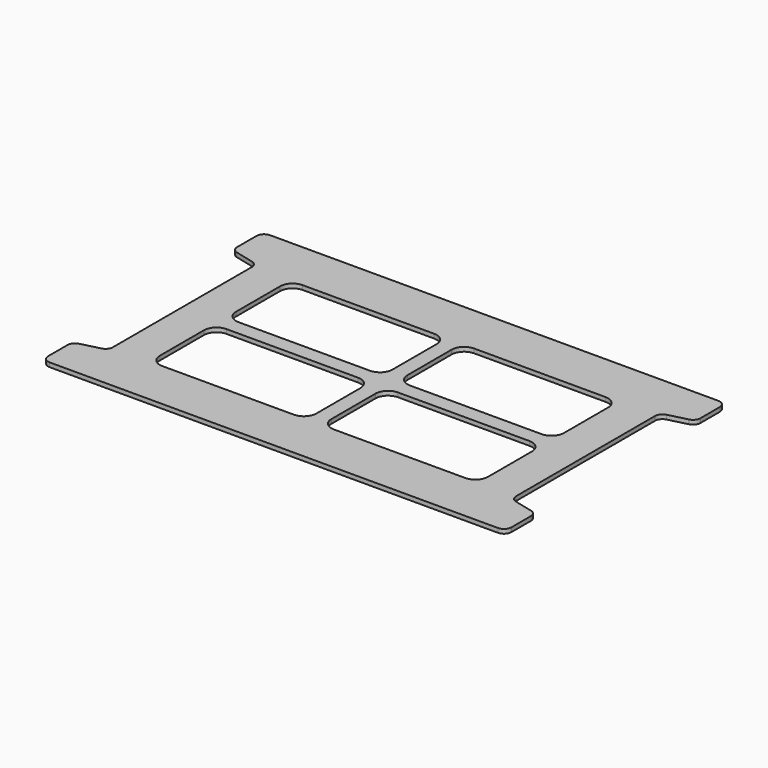
from build123d import *

# Parameters (mm, degrees)
F1_DEPTH = 1.7
F2_R     = 3
F3_W     = 62.5
F3_H     = 32
F4_DEPTH = 1.701
F5_R     = 5


with BuildPart() as f1:
    # F0 (on Top) → F1 (new body)
    with BuildSketch(Plane.XY):
        Polygon((100.0762677759, 54.24722471), (-84.9237322241, 54.24722471), (-84.9237322241, 39.24722471), (-72.9237322241, 39.24722471), (-72.9237322241, 36.24722471), (-72.9237322241, -37.75277529), (-72.9237322241, -40.75277529), (-84.9237322241, -40.75277529), (-84.9237322241, -55.75277529), (100.0762677759, -55.75277529), (100.0762677759, -40.75277529), (88.0762677759, -37.75277529), (88.0762677759, 36.24722471), (88.0762677759, 39.24722471), (100.0762677759, 39.24722471), align=None)
        Polygon((88.0762677759, 36.24722471), (100.0762677759, 39.24722471), (88.0762677759, 39.24722471), align=None)
        Polygon((-72.9237322241, 39.24722471), (-84.9237322241, 39.24722471), (-72.9237322241, 36.24722471), align=None)
        Polygon((-72.9237322241, -40.75277529), (-72.9237322241, -37.75277529), (-84.9237322241, -40.75277529), align=None)
    extrude(amount=F1_DEPTH)

    # F2
    f2_edges = [f1.edges().sort_by_distance(p)[0] for p in [
        (-72.923732, -37.752775, 0.85),
        (-72.923732, 36.247225, 0.85),
        (-84.923732, 39.247225, 0.85),
        (-84.923732, -40.752775, 0.85),
        (88.076268, 36.247225, 0.85),
        (100.076268, 39.247225, 0.85),
        (-84.923732, -55.752775, 0.85),
        (-84.923732, 54.247225, 0.85),
        (100.076268, 54.247225, 0.85),
        (100.076268, -55.752775, 0.85),
        (100.076268, -40.752775, 0.85),
        (88.076268, -37.752775, 0.85),
    ]]
    fillet(f2_edges, radius=F2_R)

    # F3 (on face) → F4 (cut, through all)
    with BuildSketch(Plane.XY.offset(1.7)):
        with Locations((-26.6737322241, 18.24722471)):
            Rectangle(F3_W, F3_H)
        with Locations((-26.6737322241, -19.75277529)):
            Rectangle(F3_W, F3_H)
        with Locations((41.8262677759, 18.24722471)):
            Rectangle(F3_W, F3_H)
        with Locations((41.8262677759, -19.75277529)):
            Rectangle(F3_W, F3_H)
    extrude(amount=-F4_DEPTH, mode=Mode.SUBTRACT)

    # F5
    f5_edges = [f1.edges().sort_by_distance(p)[0] for p in [
        (-57.923732, 34.247225, 0.85),
        (4.576268, 2.247225, 0.85),
        (73.076268, -35.752775, 0.85),
        (10.576268, -35.752775, 0.85),
        (10.576268, 2.247225, 0.85),
        (10.576268, -3.752775, 0.85),
        (10.576268, 34.247225, 0.85),
        (-57.923732, -3.752775, 0.85),
        (4.576268, -3.752775, 0.85),
        (73.076268, -3.752775, 0.85),
        (4.576268, -35.752775, 0.85),
        (-57.923732, -35.752775, 0.85),
        (4.576268, 34.247225, 0.85),
        (-57.923732, 2.247225, 0.85),
        (73.076268, 34.247225, 0.85),
        (73.076268, 2.247225, 0.85),
    ]]
    fillet(f5_edges, radius=F5_R)


solid = f1.part
